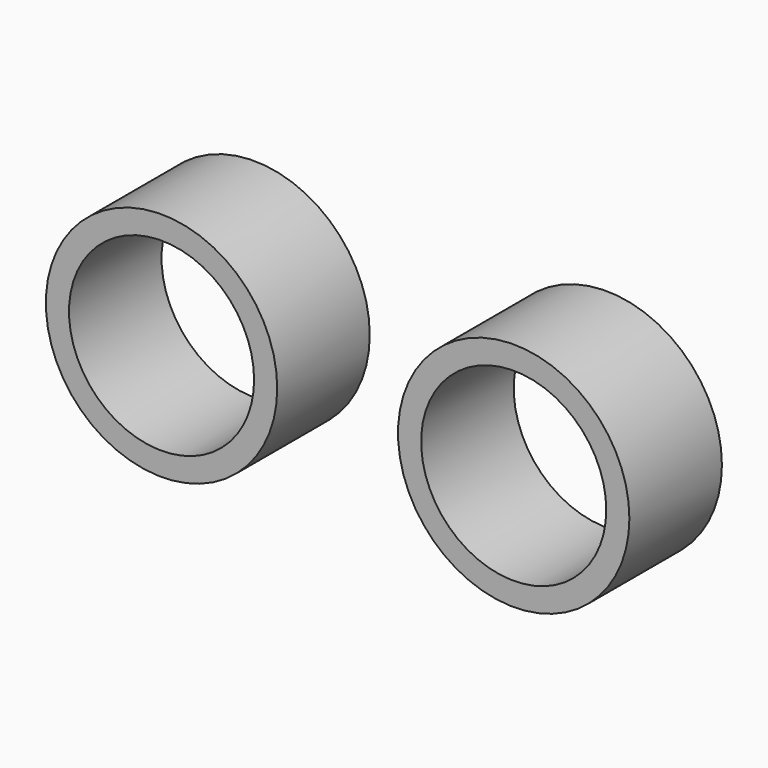
from build123d import *

# Parameters (mm, degrees)
F0_R     = 25
F0_R_2   = 20
F1_DEPTH = 25


# Not quite as in the source:
# - the program builds the solid bodies; features that only make, move or delete a surface that nothing else refers to are left out


with BuildPart() as f1:
    # F0 (on Front) → F1 (new body)
    with BuildSketch(Plane.XZ):
        with Locations((-36.9110533473, 0)):
            Circle(F0_R)
        with Locations((-36.9110533473, 0)):
            Circle(F0_R_2, mode=Mode.SUBTRACT)
    extrude(amount=F1_DEPTH)


with BuildPart() as f1b:
    # F0 (on Front) → F1, piece 2 (new body)
    with BuildSketch(Plane.XZ):
        with Locations((39.197404974, 0)):
            Circle(F0_R)
        with Locations((39.197404974, 0)):
            Circle(F0_R_2, mode=Mode.SUBTRACT)
    extrude(amount=F1_DEPTH)


solid = Compound([f1.part, f1b.part])
